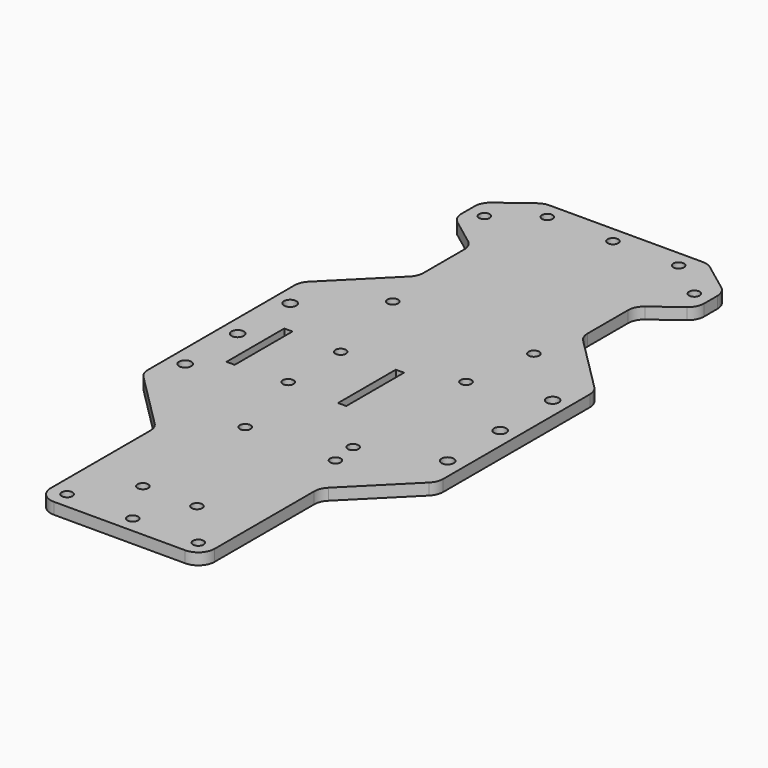
from build123d import *

# Parameters (mm, degrees)
F0_R     = 1.625
F0_R_2   = 1.875
F0_W     = 2.5
F0_H     = 22
F1_DEPTH = 3.5
F2_R     = 5


# Not quite as in the source:
# - a feature names something its author has since deleted; it is built from what else it names


with BuildPart() as f1:
    # F0 (on Top) → F1 (new body)
    with BuildSketch(Plane.XY):
        with BuildLine():
            Line((-25, 52), (-45, 32))
            Line((-45, 32), (-45, -28))
            Line((-45, -28), (-25, -48))
            Line((-25, -48), (-25, -88))
            ThreePointArc((-25, -88), (-23.5355339059, -91.5355339059), (-20, -93))
            Line((-20, -93), (20, -93))
            ThreePointArc((20, -93), (23.5355339059, -91.5355339059), (25, -88))
            Line((25, -88), (25, -48))
            Line((25, -48), (45, -28))
            Line((45, -28), (45, 32))
            Line((45, 32), (25, 52))
            Line((25, 52), (25, 72))
            Line((25, 72), (37, 81))
            Line((37, 81), (37, 91))
            Line((37, 91), (25, 100))
            Line((25, 100), (-25, 100))
            Line((-25, 100), (-37, 91))
            Line((-37, 91), (-37, 81))
            Line((-37, 81), (-25, 72))
            Line((-25, 72), (-25, 52))
        make_face()
        with Locations((-20, -88)):
            Circle(F0_R, mode=Mode.SUBTRACT)
        with Locations((-8.5, -73.5)):
            Circle(F0_R, mode=Mode.SUBTRACT)
        with Locations((-40, -18)):
            Circle(F0_R_2, mode=Mode.SUBTRACT)
        with Locations((-40, 2)):
            Circle(F0_R_2, mode=Mode.SUBTRACT)
        with Locations((-31.75, 0)):
            Rectangle(F0_W, F0_H, mode=Mode.SUBTRACT)
        with Locations((-8.5, -34.5)):
            Circle(F0_R, mode=Mode.SUBTRACT)
        with Locations((-15, -10)):
            Circle(F0_R, mode=Mode.SUBTRACT)
        with Locations((0, -88)):
            Circle(F0_R, mode=Mode.SUBTRACT)
        with Locations((8, -73.5)):
            Circle(F0_R, mode=Mode.SUBTRACT)
        with Locations((20, -88)):
            Circle(F0_R, mode=Mode.SUBTRACT)
        with Locations((19, -34.5)):
            Circle(F0_R, mode=Mode.SUBTRACT)
        with Locations((18, -26.5)):
            Circle(F0_R, mode=Mode.SUBTRACT)
        with Locations((2.25, 0)):
            Rectangle(F0_W, F0_H, mode=Mode.SUBTRACT)
        with Locations((40, -18)):
            Circle(F0_R_2, mode=Mode.SUBTRACT)
        with Locations((40, 2)):
            Circle(F0_R_2, mode=Mode.SUBTRACT)
        with Locations((-40, 22)):
            Circle(F0_R_2, mode=Mode.SUBTRACT)
        with Locations((-15, 10)):
            Circle(F0_R, mode=Mode.SUBTRACT)
        with Locations((-21.5, 38)):
            Circle(F0_R, mode=Mode.SUBTRACT)
        with Locations((-32, 86)):
            Circle(F0_R, mode=Mode.SUBTRACT)
        with Locations((-20, 95)):
            Circle(F0_R, mode=Mode.SUBTRACT)
        with Locations((18, 16.5)):
            Circle(F0_R, mode=Mode.SUBTRACT)
        with Locations((21.5, 38)):
            Circle(F0_R, mode=Mode.SUBTRACT)
        with Locations((40, 22)):
            Circle(F0_R_2, mode=Mode.SUBTRACT)
        with Locations((0, 95)):
            Circle(F0_R, mode=Mode.SUBTRACT)
        with Locations((20, 95)):
            Circle(F0_R, mode=Mode.SUBTRACT)
        with Locations((32, 86)):
            Circle(F0_R, mode=Mode.SUBTRACT)
    extrude(amount=F1_DEPTH)

    # F2
    f2_edges = [f1.edges().sort_by_distance(p)[0] for p in [
        (-45, -28, 1.75),
        (-25, -48, 1.75),
        (25, -48, 1.75),
        (45, -28, 1.75),
        (45, 32, 1.75),
        (25, 52, 1.75),
        (25, 72, 1.75),
        (-25, 52, 1.75),
        (-45, 32, 1.75),
        (-25, 72, 1.75),
        (-37, 81, 1.75),
        (-37, 91, 1.75),
        (-25, 100, 1.75),
        (25, 100, 1.75),
        (37, 91, 1.75),
        (37, 81, 1.75),
    ]]
    fillet(f2_edges, radius=F2_R)


solid = f1.part
